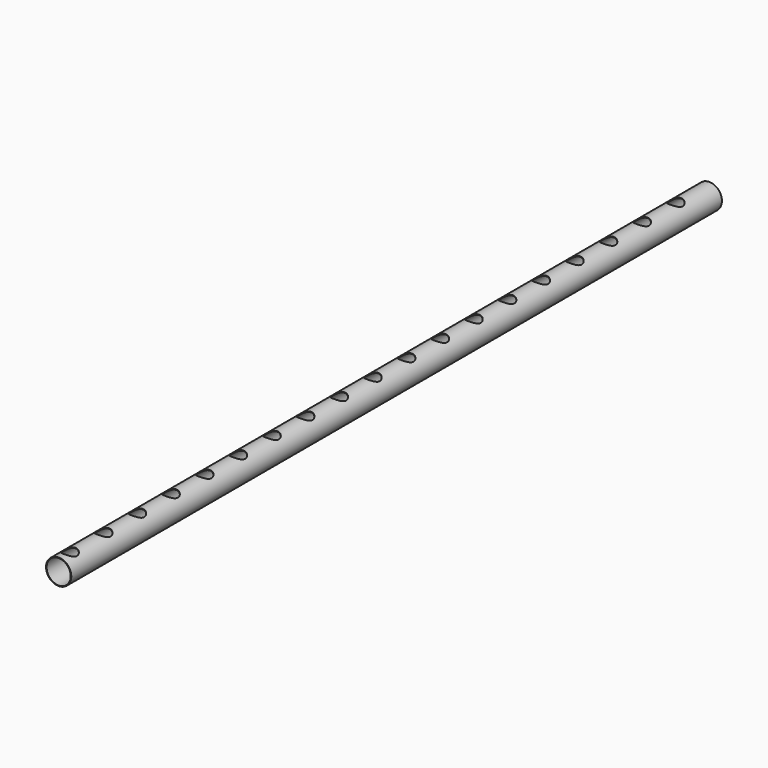
from build123d import *

# Parameters (mm, degrees)
F0_R     = 45
F0_R_2   = 43
F1_DEPTH = 1450
F4_D     = 50
F4_DEPTH = 50
F4_TIP   = 15.0215154757


# Not quite as in the source:
# - a feature names something its author has since deleted; it is built from what else it names


with BuildPart() as f1:
    # F0 (on Front) → F1 (new body, symmetric)
    with BuildSketch(Plane.XZ):
        Circle(F0_R)
        Circle(F0_R_2, mode=Mode.SUBTRACT)
    extrude(amount=F1_DEPTH, both=True)

    # F4
    with Locations(Plane.XY.offset(45)):
        with Locations((0, -1400), (0, -1250), (0, -1100), (0, -950), (0, -800), (0, -650), (0, -500), (0, -350), (0, -200), (0, -50), (0, 100), (0, 250), (0, 400), (0, 550), (0, 700), (0, 850), (0, 1000), (0, 1150), (0, 1300)):
            Hole(F4_D / 2, depth=F4_DEPTH)
            with Locations((0, 0, -(F4_DEPTH + F4_TIP / 2))):  # 118° drill point
                Cone(0, F4_D / 2, F4_TIP, mode=Mode.SUBTRACT)


solid = f1.part
